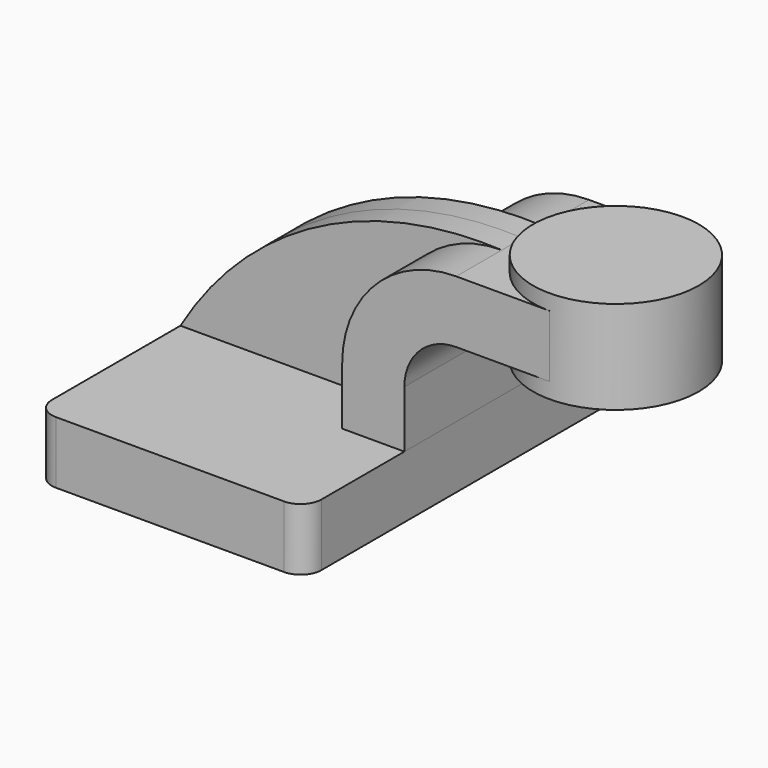
from build123d import *

# Parameters (mm, degrees)
F1_DEPTH = 63.5
F0_W     = 25.4
F0_H     = 19.05
F2_DEPTH = 25.4
F3_DEPTH = 7.9375
F5_R     = 6.35


# Not quite as in the source:
# - a feature names something its author has since deleted; it is built from what else it names


with BuildPart() as f1:
    # F0 (on Front) → F1 (new body, symmetric)
    with BuildSketch(Plane.XZ):
        Polygon((-41.275, -9.525), (41.275, -9.525), (41.275, 9.525), (22.225, 9.525), (-41.275, 9.525), align=None)
    extrude(amount=F1_DEPTH, both=True)

    # F5
    f5_edges = [f1.edges().sort_by_distance(p)[0] for p in [
        (41.275, -63.5, 0),
        (-41.275, -63.5, 0),
        (41.275, 63.5, 0),
        (-41.275, 63.5, 0),
    ]]
    fillet(f5_edges, radius=F5_R)


with BuildPart() as f2:
    # F0 (on Front) → F2 (new body, symmetric)
    with BuildSketch(Plane.XZ):
        with BuildLine():
            Line((22.225, 9.525), (41.275, 9.525))
            Line((41.275, 9.525), (41.275, 27.0002))
            ThreePointArc((41.275, 27.0002), (45.9246798487, 38.2255201513), (57.15, 42.8752))
            Line((57.15, 42.8752), (60.325, 42.8752))
            Line((60.325, 42.8752), (60.325, 61.9252))
            Line((60.325, 61.9252), (57.15, 61.9252))
            ThreePointArc((57.15, 61.9252), (32.4542956671, 51.6959043329), (22.225, 27.0002))
            Line((22.225, 27.0002), (22.225, 9.525))
        make_face()
        with Locations((73.025, 52.4002)):
            Rectangle(F0_W, F0_H)
    extrude(amount=F2_DEPTH, both=True)


with BuildPart() as f3:
    # F0 (on Front) → F3 (new body, symmetric)
    with BuildSketch(Plane.XZ):
        with BuildLine():
            add(Edge.make_bspline(
                [(-41.275, 9.525), (-20.5563157797, 44.6057990193), (15.8763434738, 63.8532415032), (57.15, 61.9252)],
                knots=[0, 0, 0, 0, 111.5045361635, 111.5045361635, 111.5045361635, 111.5045361635], degree=3))
            Line((-41.275, 9.525), (22.225, 9.525))
            Line((22.225, 9.525), (22.225, 27.0002))
            ThreePointArc((22.225, 27.0002), (32.4542956671, 51.6959043329), (57.15, 61.9252))
        make_face()
    extrude(amount=F3_DEPTH, both=True)


with BuildPart() as f4:
    # F0 (on Front) → F4 (revolve)
    with BuildSketch(Plane.XZ):
        Polygon((85.725, 66.675), (85.725, 61.9252), (85.725, 42.8752), (85.725, 38.1), (111.125, 38.1), (111.125, 66.675), align=None)
    revolve(axis=Axis((85.725, 0, 52.3875), (0, 0, 1)))


solid = Compound([f1.part, f2.part, f3.part, f4.part])
